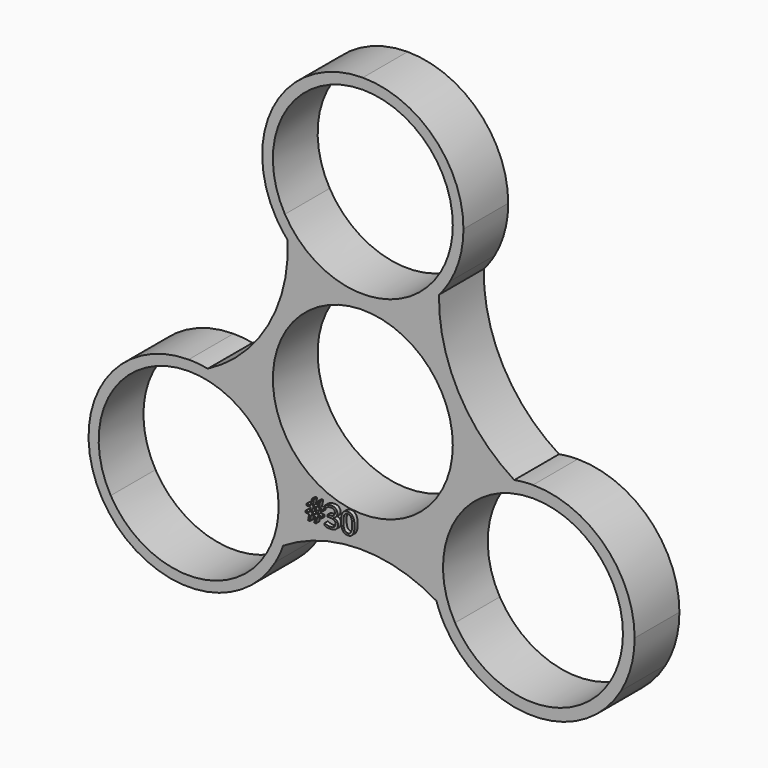
from build123d import *

# Parameters (mm, degrees)
F0_R         = 11.25
F1_DEPTH     = 7
F2_TEXT_SIZE = 3.5731749466
F3_DEPTH     = 0.5


# Not quite as in the source:
# - Text() gives the source's letters only with a copy of the font that has no kerning and outlines rounded to 1/6400 em; it was checked with that copy


with BuildPart() as f1:
    # F0 (on Front) → F1 (new body)
    with BuildSketch(Plane.XZ):
        with BuildLine():
            ThreePointArc((-9.4060207617, 29.6987205043), (-9.5238300134, 31.0708957589), (-9.7427857926, 32.4306024611))
            Line((-9.7427857926, 32.4306024611), (-10.8964685544, 31.764523408))
            ThreePointArc((-10.8964685544, 31.764523408), (-10.2036588299, 30.693805867), (-9.4060207617, 29.6987205043))
        make_face()
        with BuildLine():
            ThreePointArc((-21.7823833227, 11.25), (-20.5709521959, 11.7273505035), (-19.39586134, 12.2882340553))
            ThreePointArc((-19.39586134, 12.2882340553), (-20.5836127452, 12.4603022626), (-21.7823833227, 12.517834612))
            Line((-21.7823833227, 12.517834612), (-21.7823833227, 11.25))
        make_face()
        with BuildLine():
            ThreePointArc((-10.9416205484, -6.258917306), (-10.4024527654, -5.2147256768), (-9.9635817277, -4.1245741877))
            ThreePointArc((-9.9635817277, -4.1245741877), (-11.0277419819, -4.8386022337), (-12.0395975301, -5.625))
            Line((-12.0395975301, -5.625), (-10.9416205484, -6.258917306))
        make_face()
        with BuildLine():
            ThreePointArc((11.5310600141, -5.625), (10.3942436659, -4.7490802883), (9.192592442, -3.9644650404))
            ThreePointArc((9.192592442, -3.9644650404), (9.6655885729, -5.1886443231), (10.2622496718, -6.3575479927))
            Line((10.2622496718, -6.3575479927), (11.5310600141, -5.625))
        make_face()
        with BuildLine():
            ThreePointArc((21.2738458067, 12.7150959854), (20.1011218116, 12.6608998239), (18.9383949317, 12.498773345))
            ThreePointArc((18.9383949317, 12.498773345), (20.0854171363, 11.8356675698), (21.2738458067, 11.25))
            Line((21.2738458067, 11.25), (21.2738458067, 12.7150959854))
        make_face()
        with BuildLine():
            Line((10.8964685544, 31.764523408), (9.7427857926, 32.4306024611))
            ThreePointArc((9.7427857926, 32.4306024611), (9.5914604742, 31.1360455172), (9.5248194529, 29.8343788904))
            ThreePointArc((9.5248194529, 29.8343788904), (10.2561501273, 30.7671124134), (10.8964685544, 31.764523408))
        make_face()
        with BuildLine():
            Line((-10.8964685544, 31.764523408), (-9.7427857926, 32.4306024611))
            ThreePointArc((-9.7427857926, 32.4306024611), (-9.7427857926, 43.6806024611), (0, 49.3056024611))
            Line((0, 49.3056024611), (0, 50.6377605673))
            ThreePointArc((0, 50.6377605673), (-10.8964685544, 44.3466815142), (-10.8964685544, 31.764523408))
        make_face()
        with BuildLine():
            ThreePointArc((11.25, 38.0556024611), (10.8666655458, 35.1438882037), (9.7427857926, 32.4306024611))
            Line((9.7427857926, 32.4306024611), (10.8964685544, 31.764523408))
            ThreePointArc((10.8964685544, 31.764523408), (12.1534314652, 34.7991003147), (12.5821581062, 38.0556024611))
            ThreePointArc((12.5821581062, 38.0556024611), (8.8969293189, 46.95253178), (0, 50.6377605673))
            Line((0, 50.6377605673), (0, 49.3056024611))
            ThreePointArc((0, 49.3056024611), (7.9549512883, 46.0105537494), (11.25, 38.0556024611))
        make_face()
        with BuildLine():
            ThreePointArc((31.0166315993, -5.625), (21.2738458067, -11.25), (11.5310600141, -5.625))
            Line((11.5310600141, -5.625), (10.2622496718, -6.3575479927))
            ThreePointArc((10.2622496718, -6.3575479927), (21.2738458067, -12.7150959854), (32.2854419417, -6.3575479927))
            Line((32.2854419417, -6.3575479927), (31.0166315993, -5.625))
        make_face()
        with BuildLine():
            Line((21.2738458067, 12.7150959854), (21.2738458067, 11.25))
            ThreePointArc((21.2738458067, 11.25), (29.2287970951, 7.9549512883), (32.5238458067, 0))
            ThreePointArc((32.5238458067, 0), (32.1405113525, -2.9117142574), (31.0166315993, -5.625))
            Line((31.0166315993, -5.625), (32.2854419417, -6.3575479927))
            ThreePointArc((32.2854419417, -6.3575479927), (33.5556854028, -3.2909090013), (33.9889417921, 0))
            ThreePointArc((33.9889417921, 0), (30.2647764015, 8.9909305947), (21.2738458067, 12.7150959854))
        make_face()
        with BuildLine():
            ThreePointArc((-31.5251691153, -5.625), (-31.5251691153, 5.625), (-21.7823833227, 11.25))
            Line((-21.7823833227, 11.25), (-21.7823833227, 12.517834612))
            ThreePointArc((-21.7823833227, 12.517834612), (-32.6231460971, 6.258917306), (-32.6231460971, -6.258917306))
            Line((-32.6231460971, -6.258917306), (-31.5251691153, -5.625))
        make_face()
        with BuildLine():
            ThreePointArc((-12.0395975301, -5.625), (-21.7823833227, -11.25), (-31.5251691153, -5.625))
            Line((-31.5251691153, -5.625), (-32.6231460971, -6.258917306))
            ThreePointArc((-32.6231460971, -6.258917306), (-21.7823833227, -12.517834612), (-10.9416205484, -6.258917306))
            Line((-10.9416205484, -6.258917306), (-12.0395975301, -5.625))
        make_face()
        with BuildLine():
            ThreePointArc((9.7427857926, 32.4306024611), (0, 26.8056024611), (-9.7427857926, 32.4306024611))
            ThreePointArc((-9.7427857926, 32.4306024611), (-9.5238300134, 31.0708957589), (-9.4060207617, 29.6987205043))
            ThreePointArc((-9.4060207617, 29.6987205043), (0.0901614202, 25.4737673991), (9.5248194529, 29.8343788904))
            ThreePointArc((9.5248194529, 29.8343788904), (9.5914604742, 31.1360455172), (9.7427857926, 32.4306024611))
        make_face()
        with BuildLine():
            ThreePointArc((21.2738458067, 11.25), (20.0854171363, 11.8356675698), (18.9383949317, 12.498773345))
            ThreePointArc((18.9383949317, 12.498773345), (10.33218712, 6.4771730795), (9.192592442, -3.9644650404))
            ThreePointArc((9.192592442, -3.9644650404), (10.3942436659, -4.7490802883), (11.5310600141, -5.625))
            ThreePointArc((11.5310600141, -5.625), (11.5310600141, 5.625), (21.2738458067, 11.25))
        make_face()
        with BuildLine():
            ThreePointArc((-9.2645487107, 0), (-12.1239602928, 7.9631054211), (-19.39586134, 12.2882340553))
            ThreePointArc((-19.39586134, 12.2882340553), (-20.5709521959, 11.7273505035), (-21.7823833227, 11.25))
            ThreePointArc((-21.7823833227, 11.25), (-13.8274320344, 7.9549512883), (-10.5323833227, 0))
            ThreePointArc((-10.5323833227, 0), (-10.915717777, -2.9117142574), (-12.0395975301, -5.625))
            ThreePointArc((-12.0395975301, -5.625), (-11.0277419819, -4.8386022337), (-9.9635817277, -4.1245741877))
            ThreePointArc((-9.9635817277, -4.1245741877), (-9.4405441759, -2.091695448), (-9.2645487107, 0))
        make_face()
        with BuildLine():
            ThreePointArc((9.5248194529, 29.8343788904), (0.0901614202, 25.4737673991), (-9.4060207617, 29.6987205043))
            ThreePointArc((-9.4060207617, 29.6987205043), (-11.8526088985, 19.5312876956), (-19.39586134, 12.2882340553))
            ThreePointArc((-19.39586134, 12.2882340553), (-12.1239602928, 7.9631054211), (-9.2645487107, 0))
            ThreePointArc((-9.2645487107, 0), (-9.4405441759, -2.091695448), (-9.9635817277, -4.1245741877))
            ThreePointArc((-9.9635817277, -4.1245741877), (-0.4079859256, -1.3535619941), (9.192592442, -3.9644650404))
            ThreePointArc((9.192592442, -3.9644650404), (10.33218712, 6.4771730795), (18.9383949317, 12.498773345))
            ThreePointArc((18.9383949317, 12.498773345), (11.9442744473, 19.9245093561), (9.5248194529, 29.8343788904))
        make_face()
        with Locations((0, 13.815285638)):
            Circle(F0_R, mode=Mode.SUBTRACT)
    extrude(amount=F1_DEPTH)

    # F2 (on face) → F3 (join)
    with BuildSketch(Plane.XZ.offset(7)):
        with Locations((-6.8558917784, 0)):
            Text('#30', F2_TEXT_SIZE, font='Open Sans', text_align=(TextAlign.LEFT, TextAlign.BOTTOM))
    extrude(amount=F3_DEPTH)


solid = f1.part
